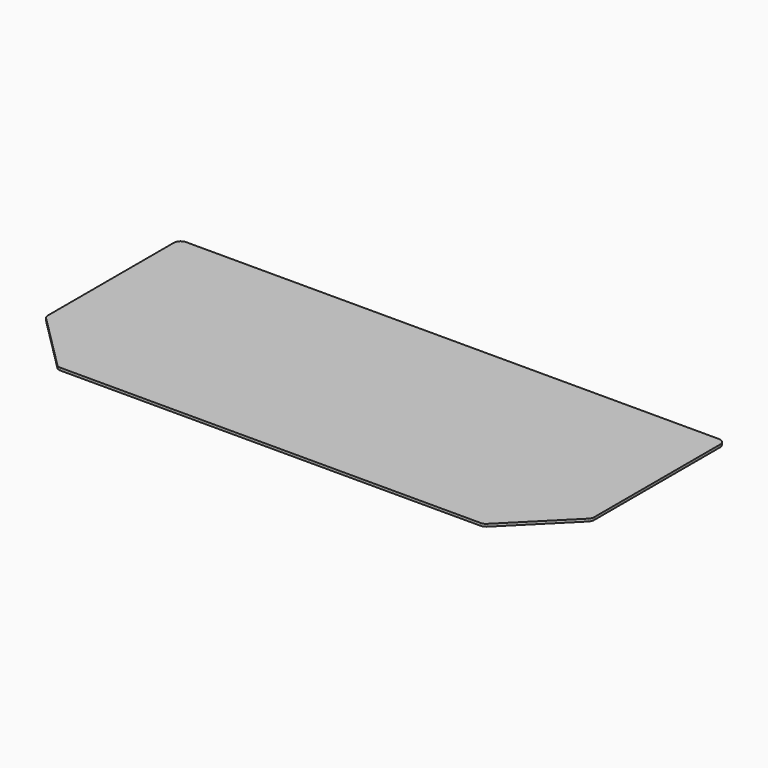
from build123d import *

# Parameters (mm, degrees)
F1_DEPTH = 1.5
F2_R     = 4


# Not quite as in the source:
# - a feature names something its author has since deleted; it is built from what else it names


with BuildPart() as f1:
    # F0 (on Top) → F1 (new body)
    with BuildSketch(Plane.XY):
        Polygon((-160.3553390593, -14.6446609407), (-125, -50), (125, -50), (160.3553390593, -14.6446609407), (160.3553390593, 83.3553390593), (-160.3553390593, 83.3553390593), align=None)
        Polygon((-118.7867965644, -35), (-145.3553390593, -8.4314575051), (-145.3553390593, 68.3553390593), (145.3553390593, 68.3553390593), (145.3553390593, -8.4314575051), (118.7867965644, -35), align=None, mode=Mode.SUBTRACT)
        Polygon((-145.3553390593, 68.3553390593), (-145.3553390593, -8.4314575051), (-118.7867965644, -35), (118.7867965644, -35), (145.3553390593, -8.4314575051), (145.3553390593, 68.3553390593), align=None)
    extrude(amount=F1_DEPTH)

    # F2
    f2_edges = [f1.edges().sort_by_distance(p)[0] for p in [
        (160.355339, -14.644661, 0.75),
        (125, -50, 0.75),
        (160.355339, 83.355339, 0.75),
        (-125, -50, 0.75),
        (-160.355339, -14.644661, 0.75),
        (-160.355339, 83.355339, 0.75),
    ]]
    fillet(f2_edges, radius=F2_R)


solid = f1.part
